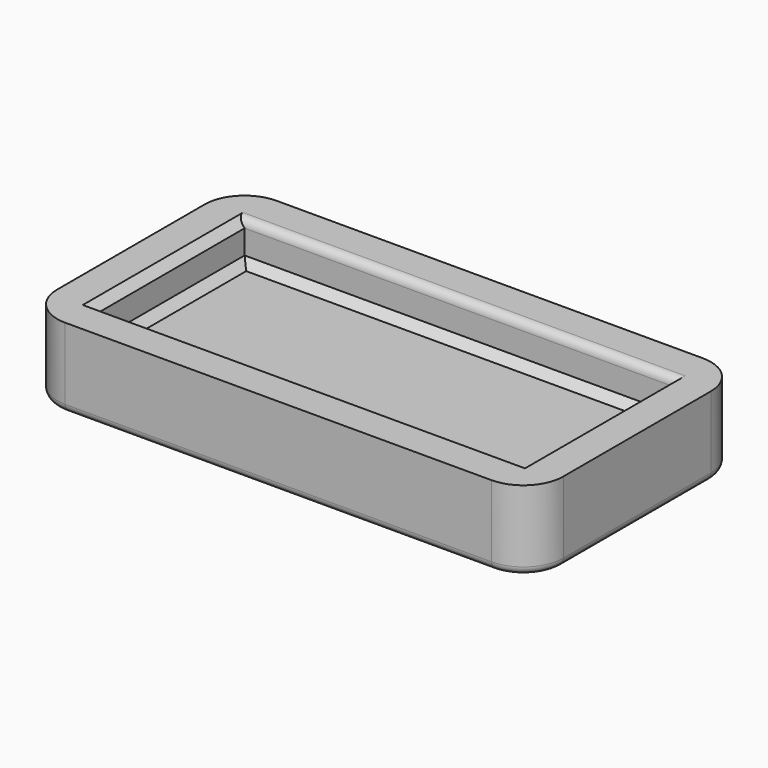
from build123d import *

# Parameters (mm, degrees)
F1_DEPTH = 25.4
F2_W     = 135.629368639
F2_H     = 58.648413825
F3_DEPTH = 12.7
F4_R     = 2.54
F5_SIZE  = 2.54


with BuildPart() as f1:
    # F0 (on Top) → F1 (new body)
    with BuildSketch(Plane.XY):
        with BuildLine():
            Line((-12.7, 0), (-148.329368639, 0))
            ThreePointArc((-148.329368639, 0), (-157.3096247601, -3.7197438789), (-161.029368639, -12.7))
            Line((-161.029368639, -12.7), (-161.029368639, -71.348413825))
            ThreePointArc((-161.029368639, -71.348413825), (-157.3096247601, -80.3286699461), (-148.329368639, -84.048413825))
            Line((-148.329368639, -84.048413825), (-12.7, -84.048413825))
            ThreePointArc((-12.7, -84.048413825), (-3.7197438789, -80.3286699461), (0, -71.348413825))
            Line((0, -71.348413825), (0, -12.7))
            ThreePointArc((0, -12.7), (-3.7197438789, -3.7197438789), (-12.7, 0))
        make_face()
    extrude(amount=F1_DEPTH)

    # F2 (on face) → F3 (cut)
    with BuildSketch(Plane.XY.offset(25.4)):
        with Locations((-80.5146843195, -42.0242069125)):
            Rectangle(F2_W, F2_H)
    extrude(amount=-F3_DEPTH, mode=Mode.SUBTRACT)

    # F4
    f4_edges = [f1.edges().sort_by_distance(p)[0] for p in [
        (-80.514684, -12.7, 25.4),
        (-80.514684, 0, 0),
        (-157.309625, -3.719744, 0),
        (-161.029369, -42.024207, 0),
        (-157.309625, -80.32867, 0),
        (-80.514684, -84.048414, 0),
        (-3.719744, -80.32867, 0),
        (0, -42.024207, 0),
        (-3.719744, -3.719744, 0),
    ]]
    fillet(f4_edges, radius=F4_R)

    # F5
    f5_edges = [f1.edges().sort_by_distance(p)[0] for p in [
        (-12.7, -42.024207, 12.7),
        (-80.514684, -12.7, 12.7),
        (-148.329369, -42.024207, 12.7),
        (-80.514684, -71.348414, 12.7),
        (-80.514684, -10.16, 25.4),
        (-148.329369, -42.024207, 25.4),
        (-80.514684, -71.348414, 25.4),
        (-12.7, -42.024207, 25.4),
    ]]
    chamfer(f5_edges, length=F5_SIZE)


solid = f1.part
